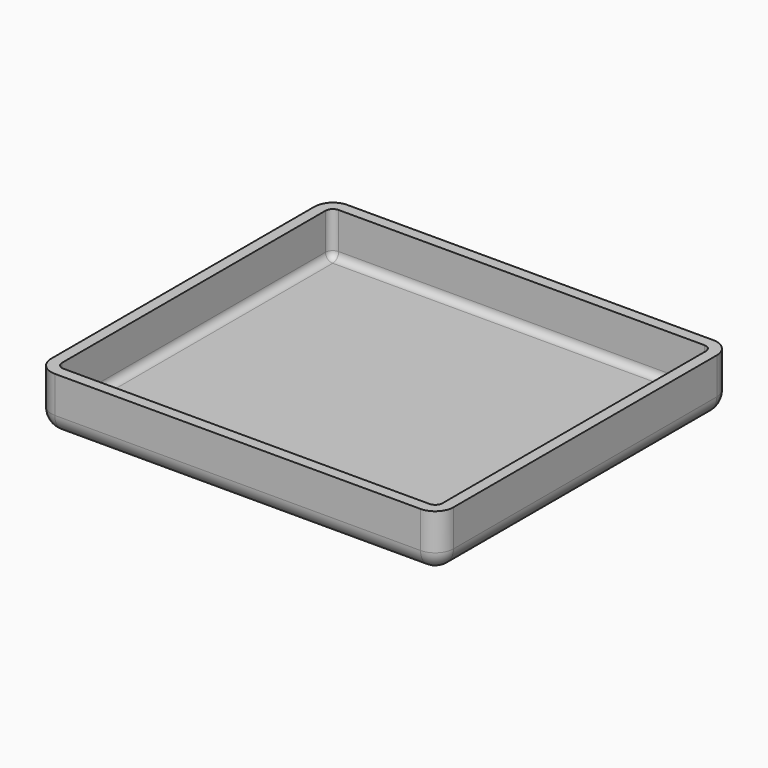
from build123d import *

# Parameters (mm, degrees)
F0_W         = 110
F0_H         = 100
F1_DEPTH     = 15
F2_R         = 5
F3_T1_DEPTH  = 22.5
F3_S5_W      = 5
F3_S5_H      = 5
F3_T6_DEPTH  = 5
F3_S11_W     = 5
F3_S11_H     = 5
F3_T12_DEPTH = 5
F3_S17_W     = 5
F3_S17_H     = 5
F3_T18_DEPTH = 5
F3_S23_W     = 5
F3_S23_H     = 5
F3_T24_DEPTH = 5
F4_T         = -3


# Not quite as in the source:
# - a fillet or chamfer that OpenCascade refuses, or shapes differently, is made with other operations: its cross-section is extruded or revolved along the edge and cut away or added


with BuildPart() as f1:
    # F0 (on Top) → F1 (new body)
    with BuildSketch(Plane.XY):
        with Locations((-55, 50)):
            Rectangle(F0_W, F0_H)
    extrude(amount=F1_DEPTH)

    # F2
    f2_edges = [f1.edges().sort_by_distance(p)[0] for p in [
        (-55, 0, 0),
        (0, 50, 0),
        (-55, 100, 0),
        (-110, 50, 0),
    ]]
    fillet(f2_edges, radius=F2_R)

    # F3: fillet of radius 5 on 4 edges, made by hand

    # F3_s2 → F3_t1 (cut)
    with BuildSketch(Plane.XY.offset(5)):
        with BuildLine():
            ThreePointArc((0, 5), (-1.4644660941, 1.4644660941), (-5, 0))
            Line((-5, 0), (0, 0))
            Line((0, 0), (0, 5))
        make_face()
        with BuildLine():
            ThreePointArc((-110, 5), (-108.5355339059, 1.4644660941), (-105, 0))
            Line((-105, 0), (-110, 0))
            Line((-110, 0), (-110, 5))
        make_face()
        with BuildLine():
            ThreePointArc((-5, 100), (-1.4644660941, 98.5355339059), (0, 95))
            Line((0, 95), (0, 100))
            Line((0, 100), (-5, 100))
        make_face()
        with BuildLine():
            ThreePointArc((-105, 100), (-108.5355339059, 98.5355339059), (-110, 95))
            Line((-110, 95), (-110, 100))
            Line((-110, 100), (-105, 100))
        make_face()
    extrude(amount=F3_T1_DEPTH, mode=Mode.SUBTRACT)


with BuildPart() as f3_tool4:
    # F3_s5 → F3_t6 (new body)
    with BuildSketch(Plane.XZ.offset(-95)):
        with Locations((-107.5, 2.5)):
            Rectangle(F3_S5_W, F3_S5_H)
    extrude(amount=-F3_T6_DEPTH)

    # F3_s7 → F3_t8 (revolve, cut)
    with BuildSketch(Plane(origin=(-105, 95, 5), x_dir=(0.7071067812, 0, 0.7071067812), z_dir=(-0.7071067812, 0, 0.7071067812))):
        with BuildLine():
            ThreePointArc((0, -5), (5, 0), (0, 5))
            Line((0, 5), (0, -5))
        make_face()
    revolve(axis=Axis((-105, 95, 5), (0, 1, 0)), mode=Mode.SUBTRACT)


with BuildPart() as f1_1:
    add(f1.part)

    # F3_t3: cut F3_tool4
    add(f3_tool4.part, mode=Mode.SUBTRACT)


with BuildPart() as f3_tool10:
    # F3_s11 → F3_t12 (new body)
    with BuildSketch(Plane.XZ.offset(-95)):
        with Locations((-2.5, 2.5)):
            Rectangle(F3_S11_W, F3_S11_H)
    extrude(amount=-F3_T12_DEPTH)

    # F3_s13 → F3_t14 (revolve, cut)
    with BuildSketch(Plane(origin=(-5, 95, 5), x_dir=(-0.7071067812, 0, 0.7071067812), z_dir=(-0.7071067812, 0, -0.7071067812))):
        with BuildLine():
            ThreePointArc((0, -5), (5, 0), (0, 5))
            Line((0, 5), (0, -5))
        make_face()
    revolve(axis=Axis((-5, 95, 5), (0, 1, 0)), mode=Mode.SUBTRACT)


with BuildPart() as f1_2:
    add(f1_1.part)

    # F3_t9: cut F3_tool10
    add(f3_tool10.part, mode=Mode.SUBTRACT)


with BuildPart() as f3_tool16:
    # F3_s17 → F3_t18 (new body)
    with BuildSketch(Plane.YZ.offset(-105)):
        with Locations((2.5, 2.5)):
            Rectangle(F3_S17_W, F3_S17_H)
    extrude(amount=-F3_T18_DEPTH)

    # F3_s19 → F3_t20 (revolve, cut)
    with BuildSketch(Plane(origin=(-105, 5, 5), x_dir=(0, 0.7071067812, 0.7071067812), z_dir=(0, -0.7071067812, 0.7071067812))):
        with BuildLine():
            ThreePointArc((0, -5), (5, 0), (0, 5))
            Line((0, 5), (0, -5))
        make_face()
    revolve(axis=Axis((-105, 5, 5), (-1, 0, 0)), mode=Mode.SUBTRACT)


with BuildPart() as f1_3:
    add(f1_2.part)

    # F3_t15: cut F3_tool16
    add(f3_tool16.part, mode=Mode.SUBTRACT)


with BuildPart() as f3_tool22:
    # F3_s23 → F3_t24 (new body)
    with BuildSketch(Plane.YZ.offset(-5)):
        with Locations((2.5, 2.5)):
            Rectangle(F3_S23_W, F3_S23_H)
    extrude(amount=F3_T24_DEPTH)

    # F3_s25 → F3_t26 (revolve, cut)
    with BuildSketch(Plane(origin=(-5, 5, 5), x_dir=(0, 0.7071067812, 0.7071067812), z_dir=(0, 0.7071067812, -0.7071067812))):
        with BuildLine():
            ThreePointArc((0, -5), (5, 0), (0, 5))
            Line((0, 5), (0, -5))
        make_face()
    revolve(axis=Axis((-5, 5, 5), (1, 0, 0)), mode=Mode.SUBTRACT)


with BuildPart() as f1_4:
    add(f1_3.part)

    # F3_t21: cut F3_tool22
    add(f3_tool22.part, mode=Mode.SUBTRACT)

    # F4
    f4_openings = [f1_4.faces().sort_by_distance(p)[0] for p in [
        (-55, 50, 15),
    ]]
    offset(amount=F4_T, openings=f4_openings)


solid = f1_4.part
